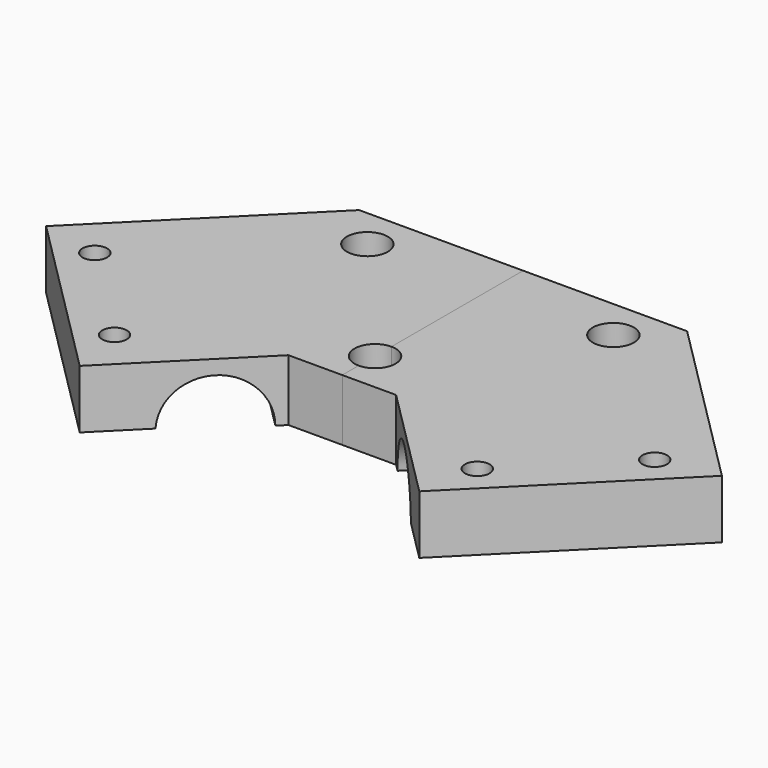
from build123d import *
from build123d import SkipClean  # not in build123d's __all__

# Parameters (mm, degrees)
F0_R      = 2.5
F1_DEPTH  = 15
F3_DEPTH  = 29
F4_R      = 1.5
F5_DEPTH  = 7.15
F6_R      = 1
F7_DEPTH  = 7.15
F10_DEPTH = 55


with BuildPart() as f1:
    # F0 (on Top) → F1 (new body)
    with BuildSketch(Plane.XY):
        with BuildLine():
            Line((0, 0), (-20, 0))
            Line((-20, 0), (-41.2132034356, -21.2132034356))
            Line((-41.2132034356, -21.2132034356), (-20.7071067812, -41.71930009))
            Line((-20.7071067812, -41.71930009), (-6.5649711575, -27.5771644663))
            Line((-6.5649711575, -27.5771644663), (0, -27.5771644663))
            Line((0, -27.5771644663), (0, -25.0771644663))
            ThreePointArc((0, -25.0771644663), (-2.5, -22.5771644663), (0, -20.0771644663))
            Line((0, -20.0771644663), (0, 0))
        make_face()
        with Locations((-15, -5)):
            Circle(F0_R, mode=Mode.SUBTRACT)
    extrude(amount=F1_DEPTH)

    # F2 (on face) → F3 (cut, through all)
    with BuildSketch(Plane(origin=(-10, 10, 0), x_dir=(-0.7071067812, -0.7071067812, 0), z_dir=(-0.7071067812, 0.7071067812, 0))):
        with BuildLine():
            Line((44.1421356237, 7.85), (36.8814735646, 7.85))
            ThreePointArc((36.8814735646, 7.85), (25.3921356237, 7.5), (36.8814735646, 7.15))
            Line((36.8814735646, 7.15), (44.1421356237, 7.15))
            Line((44.1421356237, 7.15), (44.1421356237, 7.85))
        make_face()
    extrude(amount=-F3_DEPTH, mode=Mode.SUBTRACT)

    # F4 (on face) → F5 (cut, through all)
    with BuildSketch(Plane.XY.offset(15)):
        with Locations((-34.1421356237, -22.627416998)):
            Circle(F4_R)
        with Locations((-22.1213203436, -34.6482322781)):
            Circle(F4_R)
    extrude(amount=-F5_DEPTH, mode=Mode.SUBTRACT)

    # F6 (on face) → F7 (cut, through all)
    with BuildSketch(Plane(origin=(0, 0, 0), x_dir=(1, 0, 0), z_dir=(0, 0, -1))):
        with Locations((-22.1213203436, 34.6482322781)):
            Circle(F6_R)
        with Locations((-34.1421356237, 22.627416998)):
            Circle(F6_R)
    extrude(amount=-F7_DEPTH, mode=Mode.SUBTRACT)

    # F8: F1 across plane


with BuildPart() as f1_1:
    add(f1.part, clean=False)
    with SkipClean():  # cleaning this boolean's faces spoils the solid; the shape is the same uncleaned
        add(f1.part.mirror(Plane.YZ), clean=False)

    # F9 (on face) → F10 (cut)
    with BuildSketch(Plane(origin=(0, 0, 0), x_dir=(-1, 0, 0), z_dir=(0, 1, 0))):
        Polygon((47.4618822336, 7.5), (-20, 7.5), (-48.8657653332, 7.5), (-48.8657653332, -7.0414701477), (47.4618822336, -7.0414701477), align=None)
    with SkipClean():  # cleaning this boolean's faces spoils the solid; the shape is the same uncleaned
        extrude(amount=-F10_DEPTH, mode=Mode.SUBTRACT)


solid = f1_1.part
